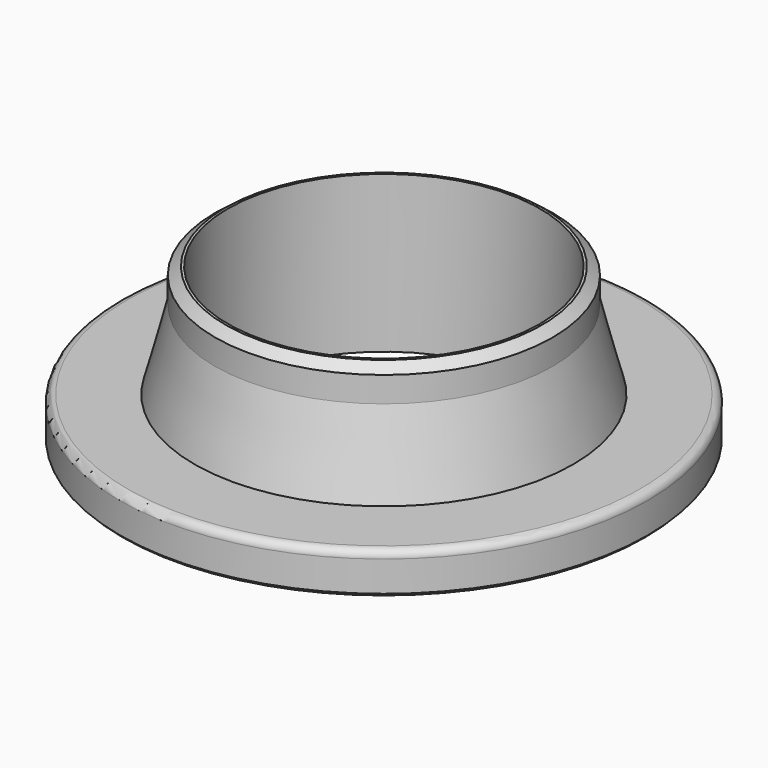
from build123d import *

# Parameters (mm, degrees)
F2_R    = 5
F3_SIZE = 2


with BuildPart() as f1:
    # F0 (on Front) → F1 (revolve)
    with BuildSketch(Plane.XZ):
        Polygon((-79.4498865843, -12.5698290182), (-79.4498865843, 89.0301709818), (-81.0498865843, 89.0301709818), (-87.6998865843, 83.9274465117), (-87.6998865843, 67.3713907599), (-101.1498865843, 15.8301709818), (-149.5498865843, 15.8301709818), (-149.5498865843, -10.9698290182), (-109.9510937929, -10.9698290182), (-109.9498865843, -12.5698290182), align=None)
    revolve(axis=Axis((21.9001134157, 0, 0.9622275829), (0, 0, -1)))

    # F2
    f2_edges = [f1.edges().sort_by_distance(p)[0] for p in [
        (193.350113, 0, 15.830171),
    ]]
    fillet(f2_edges, radius=F2_R)

    # F3
    f3_edges = [f1.edges().sort_by_distance(p)[0] for p in [
        (193.350113, 0, -10.969829),
    ]]
    chamfer(f3_edges, length=F3_SIZE)


solid = f1.part
